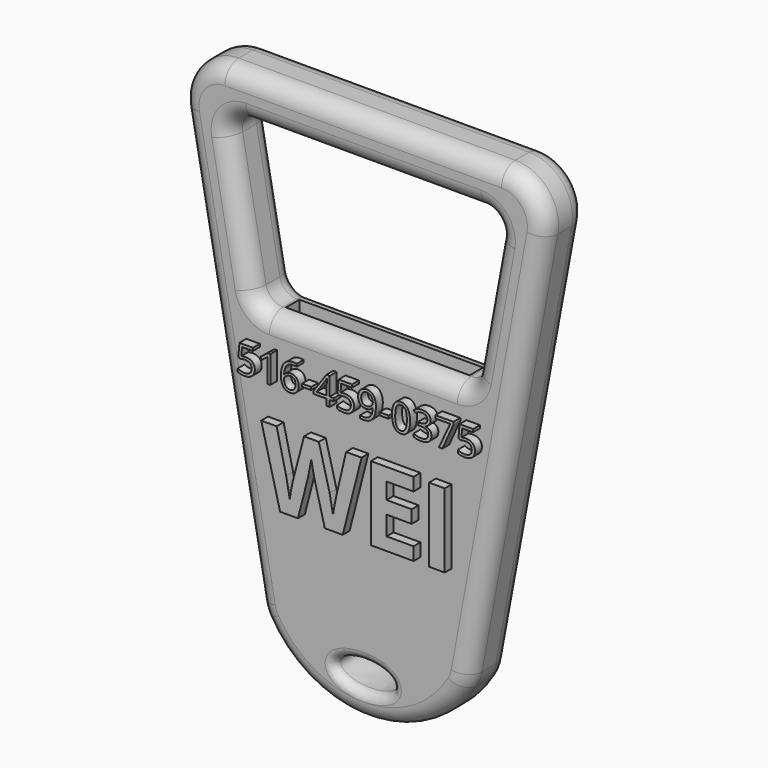
from build123d import *

# Parameters (mm, degrees)
F1_DEPTH     = 6
F2_R         = 5
F4_R         = 2
F5_DEPTH     = 15
F6_R         = 1
F7_TEXT_SIZE = 12.0023868383
F8_DEPTH     = 1
F9_TEXT_SIZE = 4.3970065023
F10_DEPTH    = 1


# Not quite as in the source:
# - Text() gives the source's letters only with a copy of the font that has no kerning and outlines rounded to 1/6400 em; it was checked with that copy


with BuildPart() as f1:
    # F0 (on Front) → F1 (new body)
    with BuildSketch(Plane.XZ):
        Polygon((22, 23.6833111547), (0, 23.6833111547), (-22, 23.6833111547), (-12, -30.3999579773), (0, -30.3999579773), (12, -30.3999579773), align=None)
        Polygon((-12.5362024197, 0), (-15.9907478742, 18.6833111547), (-4.5457669822, 18.6833111547), (15.9907478742, 18.6833111547), (12.5362024197, 0), align=None, mode=Mode.SUBTRACT)
        with BuildLine():
            ThreePointArc((-12, -30.3999579773), (0, -37.8549291284), (12, -30.3999579773))
            Line((12, -30.3999579773), (0, -30.3999579773))
            Line((0, -30.3999579773), (-12, -30.3999579773))
        make_face()
        with BuildLine():
            add(Edge.make_bspline(
                [(3.4030418817, -33.2950651646), (3.4030418817, -30.663743683), (-1.7015209408, -31.9794044238), (-6.8060837633, -33.2950651646), (-1.7015209408, -34.6107259053), (3.4030418817, -35.9263866461), (3.4030418817, -33.2950651646)],
                knots=[0, 0, 0, 2.0943951024, 2.0943951024, 4.1887902048, 4.1887902048, 6.2831853072, 6.2831853072, 6.2831853072], degree=2, weights=[1, 0.5, 1, 0.5, 1, 0.5, 1]))
        make_face(mode=Mode.SUBTRACT)
    extrude(amount=F1_DEPTH)

    # F2
    f2_edges = [f1.edges().sort_by_distance(p)[0] for p in [
        (-22, -3, 23.683311),
        (22, -3, 23.683311),
        (-12, -3, -30.399958),
        (12, -3, -30.399958),
    ]]
    fillet(f2_edges, radius=F2_R)

    # F4
    f4_edges = [f1.edges().sort_by_distance(p)[0] for p in [
        (0, -6, 23.683311),
        (-16.524404, 0, -5.930501),
        (-20.907409, -3, 17.77422),
        (-12.1414, -3, -29.635223),
        (-16.524404, -6, -5.930501),
        (-12.536202, -3, 0),
        (12.536202, -3, 0),
        (-15.990748, -3, 18.683311),
        (15.990748, -3, 18.683311),
        (0, 0, 18.683311),
        (0, -6, 18.683311),
        (0, 0, 23.683311),
        (19.834278, 0, 21.881322),
        (-19.834278, 0, 21.881322),
        (16.524404, 0, -5.930501),
        (11.908383, 0, -30.47641),
        (-11.908383, 0, -30.47641),
        (0, 0, -37.854929),
        (14.263475, 0, 9.341656),
        (0, 0, 0),
        (-14.263475, 0, 9.341656),
        (19.834278, -6, 21.881322),
        (-19.834278, -6, 21.881322),
        (16.524404, -6, -5.930501),
        (11.908383, -6, -30.47641),
        (-11.908383, -6, -30.47641),
        (0, -6, -37.854929),
        (14.263475, -6, 9.341656),
        (0, -6, 0),
        (-14.263475, -6, 9.341656),
    ]]
    fillet(f4_edges, radius=F4_R)

    # F3 (on face) → F5 (cut)
    with BuildSketch(Plane.XY):
        Polygon((10.625, -1.9439970143), (0, -1.9439970143), (-10.625, -1.9439970143), (-10.625, -3.8939970143), (0, -3.8939970143), (10.625, -3.8939970143), align=None)
    extrude(amount=-F5_DEPTH, mode=Mode.SUBTRACT)

    # F6
    f6_edges = [f1.edges().sort_by_distance(p)[0] for p in [
        (-3.403042, -6, -33.295064),
        (-3.403042, 0, -33.295064),
    ]]
    fillet(f6_edges, radius=F6_R)

    # F7 (on face) → F8 (join)
    with BuildSketch(Plane.XZ.offset(6)):
        with Locations((-11, -18.9458546846)):
            Text('WEI', F7_TEXT_SIZE, font='Open Sans', font_style=FontStyle.BOLD, text_align=(TextAlign.LEFT, TextAlign.BOTTOM))
    extrude(amount=F8_DEPTH)


with BuildPart() as f10:
    # F9 (on face) → F10 (new body)
    with BuildSketch(Plane.XZ.offset(6)):
        with Locations((-14, -6.4171491559)):
            Text('516-459-0375', F9_TEXT_SIZE, font='Open Sans', text_align=(TextAlign.LEFT, TextAlign.BOTTOM))
    extrude(amount=F10_DEPTH)


with BuildPart() as f11_1:
    # F11: copy of F1
    add(f1.part)


solid = Compound([f1.part, f10.part, f11_1.part])
